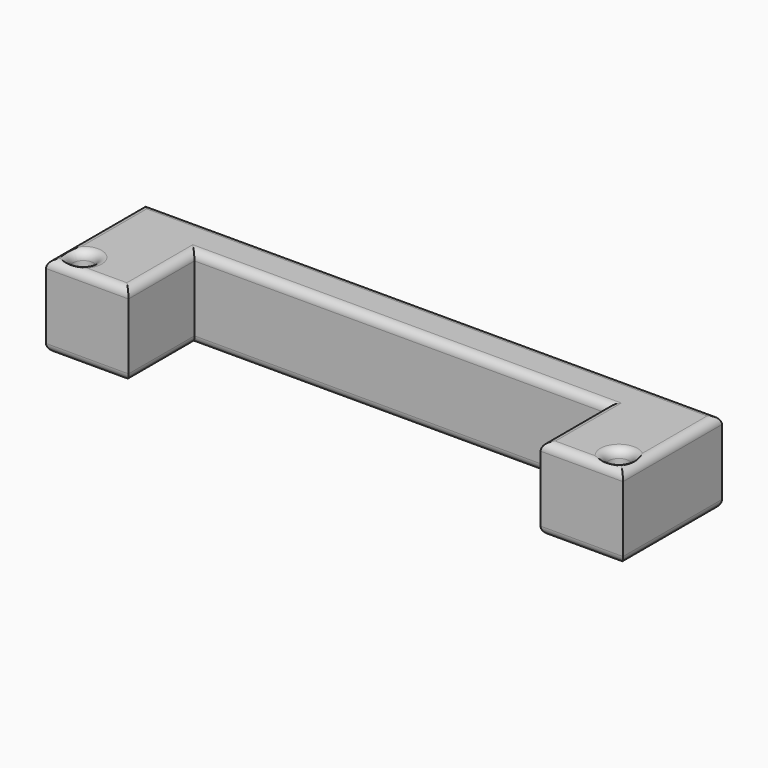
from build123d import *

# Parameters (mm, degrees)
F1_DEPTH     = 20
F3_D         = 5
F5_T1_DEPTH  = 150
F5_T3_DEPTH  = 40
F5_T5_DEPTH  = 30
F5_T7_DEPTH  = 25
F5_T9_DEPTH  = 100
F5_T11_DEPTH = 30
F5_T25_DEPTH = 105
F5_T29_DEPTH = 30
F5_T36_DEPTH = 30
F5_T40_DEPTH = 105
F5_T47_DEPTH = 30
F5_T51_DEPTH = 105
F5_T58_DEPTH = 105
F5_T62_DEPTH = 30


# Not quite as in the source:
# - a fillet or chamfer that OpenCascade refuses, or shapes differently, is made with other operations: its cross-section is extruded or revolved along the edge and cut away or added


with BuildPart() as f1:
    # F0 (on Top) → F1 (new body)
    with BuildSketch(Plane.XY):
        Polygon((0, 30), (0, 20), (50, 20), (50, 0), (70, 0), (70, 30), align=None)
    extrude(amount=F1_DEPTH)

    # F3 (through all)
    with Locations(Plane.XY.offset(20)):
        with Locations((65, 5)):
            Hole(F3_D / 2)

    # F4: F1 across face


with BuildPart() as f1_1:
    add(f1.part)
    add(f1.part.mirror(Plane(origin=(0, 25, 10), x_dir=(0, -1, 0), z_dir=(-1, 0, 0))))

    # F5: fillet of radius 2 on 20 edges, made by hand

    # F5_s2 → F5_t1 (cut)
    with BuildSketch(Plane.YZ.offset(-75)):
        with BuildLine():
            ThreePointArc((30, 18), (29.4142135624, 19.4142135624), (28, 20))
            Line((28, 20), (30, 20))
            Line((30, 20), (30, 18))
        make_face()
        with BuildLine():
            ThreePointArc((30, 2), (29.4142135624, 0.5857864376), (28, 0))
            Line((28, 0), (30, 0))
            Line((30, 0), (30, 2))
        make_face()
    extrude(amount=F5_T1_DEPTH, mode=Mode.SUBTRACT)

    # F5_s4 → F5_t3 (cut)
    with BuildSketch(Plane.XZ.offset(-35)):
        with BuildLine():
            ThreePointArc((-70, 18), (-69.4142135624, 19.4142135624), (-68, 20))
            Line((-68, 20), (-70, 20))
            Line((-70, 20), (-70, 18))
        make_face()
        with BuildLine():
            ThreePointArc((68, 20), (69.4142135624, 19.4142135624), (70, 18))
            Line((70, 18), (70, 20))
            Line((70, 20), (68, 20))
        make_face()
        with BuildLine():
            ThreePointArc((-68, 0), (-69.4142135624, 0.5857864376), (-70, 2))
            Line((-70, 2), (-70, 0))
            Line((-70, 0), (-68, 0))
        make_face()
        with BuildLine():
            ThreePointArc((68, 0), (69.4142135624, 0.5857864376), (70, 2))
            Line((70, 2), (70, 0))
            Line((70, 0), (68, 0))
        make_face()
    extrude(amount=F5_T3_DEPTH, mode=Mode.SUBTRACT)

    # F5_s6 → F5_t5 (cut)
    with BuildSketch(Plane.YZ.offset(-75)):
        with BuildLine():
            ThreePointArc((0, 18), (0.5857864376, 19.4142135624), (2, 20))
            Line((2, 20), (0, 20))
            Line((0, 20), (0, 18))
        make_face()
        with BuildLine():
            ThreePointArc((2, 0), (0.5857864376, 0.5857864376), (0, 2))
            Line((0, 2), (0, 0))
            Line((0, 0), (2, 0))
        make_face()
    extrude(amount=F5_T5_DEPTH, mode=Mode.SUBTRACT)

    # F5_s8 → F5_t7 (cut)
    with BuildSketch(Plane.XZ.offset(-20)):
        with BuildLine():
            ThreePointArc((-50, 18), (-50.5857864376, 19.4142135624), (-52, 20))
            Line((-52, 20), (-50, 20))
            Line((-50, 20), (-50, 18))
        make_face()
        with BuildLine():
            ThreePointArc((50, 18), (50.5857864376, 19.4142135624), (52, 20))
            Line((52, 20), (50, 20))
            Line((50, 20), (50, 18))
        make_face()
        with BuildLine():
            ThreePointArc((-52, 0), (-50.5857864376, 0.5857864376), (-50, 2))
            Line((-50, 2), (-50, 0))
            Line((-50, 0), (-52, 0))
        make_face()
        with BuildLine():
            ThreePointArc((52, 0), (50.5857864376, 0.5857864376), (50, 2))
            Line((50, 2), (50, 0))
            Line((50, 0), (52, 0))
        make_face()
    extrude(amount=F5_T7_DEPTH, mode=Mode.SUBTRACT)

    # F5_s10 → F5_t9 (cut)
    with BuildSketch(Plane.YZ.offset(-50)):
        with BuildLine():
            ThreePointArc((20, 18), (20.5857864376, 19.4142135624), (22, 20))
            Line((22, 20), (20, 20))
            Line((20, 20), (20, 18))
        make_face()
        with BuildLine():
            ThreePointArc((22, 0), (20.5857864376, 0.5857864376), (20, 2))
            Line((20, 2), (20, 0))
            Line((20, 0), (22, 0))
        make_face()
    extrude(amount=F5_T9_DEPTH, mode=Mode.SUBTRACT)

    # F5_s12 → F5_t11 (cut)
    with BuildSketch(Plane.YZ.offset(45)):
        with BuildLine():
            ThreePointArc((0, 18), (0.5857864376, 19.4142135624), (2, 20))
            Line((2, 20), (0, 20))
            Line((0, 20), (0, 18))
        make_face()
        with BuildLine():
            ThreePointArc((2, 0), (0.5857864376, 0.5857864376), (0, 2))
            Line((0, 2), (0, 0))
            Line((0, 0), (2, 0))
        make_face()
    extrude(amount=F5_T11_DEPTH, mode=Mode.SUBTRACT)

    # F5_s13 → F5_t14 (revolve, cut)
    with BuildSketch(Plane.XZ.offset(-5)):
        with BuildLine():
            ThreePointArc((67.5, 18), (68.0857864376, 19.4142135624), (69.5, 20))
            Line((69.5, 20), (67.5, 20))
            Line((67.5, 20), (67.5, 18))
        make_face()
    revolve(axis=Axis((65, 5, 20), (0, 0, 1)), mode=Mode.SUBTRACT)

    # F5_s15 → F5_t16 (revolve, cut)
    with BuildSketch(Plane.XZ.offset(-5)):
        with BuildLine():
            ThreePointArc((-67.5, 18), (-68.0857864376, 19.4142135624), (-69.5, 20))
            Line((-69.5, 20), (-67.5, 20))
            Line((-67.5, 20), (-67.5, 18))
        make_face()
    revolve(axis=Axis((-65, 5, 20), (0, 0, -1)), mode=Mode.SUBTRACT)

    # F5_s17 → F5_t18 (revolve, cut)
    with BuildSketch(Plane.XZ.offset(-5)):
        with BuildLine():
            ThreePointArc((69.5, 0), (68.0857864376, 0.5857864376), (67.5, 2))
            Line((67.5, 2), (67.5, 0))
            Line((67.5, 0), (69.5, 0))
        make_face()
    revolve(axis=Axis((65, 5, 0), (0, 0, 1)), mode=Mode.SUBTRACT)

    # F5_s19 → F5_t20 (revolve, cut)
    with BuildSketch(Plane.XZ.offset(-5)):
        with BuildLine():
            ThreePointArc((-69.5, 0), (-68.0857864376, 0.5857864376), (-67.5, 2))
            Line((-67.5, 2), (-67.5, 0))
            Line((-67.5, 0), (-69.5, 0))
        make_face()
    revolve(axis=Axis((-65, 5, 0), (0, 0, -1)), mode=Mode.SUBTRACT)


with BuildPart() as f5_tool23:
    # F5_s24 → F5_t25 (new body)
    with BuildSketch(Plane.YZ.offset(-55)):
        with BuildLine():
            ThreePointArc((20, 18), (20.5857864376, 19.4142135624), (22, 20))
            Line((22, 20), (20, 20))
            Line((20, 20), (20, 18))
        make_face()
    extrude(amount=F5_T25_DEPTH)

    split(bisect_by=Plane.YZ.offset(-50), keep=Keep.BOTTOM)


with BuildPart() as f5_tool27:
    # F5_s28 → F5_t29 (new body)
    with BuildSketch(Plane.XZ.offset(-25)):
        with BuildLine():
            ThreePointArc((-50, 18), (-50.5857864376, 19.4142135624), (-52, 20))
            Line((-52, 20), (-50, 20))
            Line((-50, 20), (-50, 18))
        make_face()
    extrude(amount=F5_T29_DEPTH)

    split(bisect_by=Plane.XZ.offset(-20), keep=Keep.BOTTOM)


with BuildPart() as f5_tool23_1:
    add(f5_tool23.part)

    # F5_t31: intersect F5_tool27
    add(f5_tool27.part, mode=Mode.INTERSECT)


with BuildPart() as f1_2:
    add(f1_1.part)

    # F5_t21: cut F5_tool23
    add(f5_tool23_1.part, mode=Mode.SUBTRACT)


with BuildPart() as f5_tool34:
    # F5_s35 → F5_t36 (new body)
    with BuildSketch(Plane.XZ.offset(-25)):
        with BuildLine():
            ThreePointArc((50, 18), (50.5857864376, 19.4142135624), (52, 20))
            Line((52, 20), (50, 20))
            Line((50, 20), (50, 18))
        make_face()
    extrude(amount=F5_T36_DEPTH)

    split(bisect_by=Plane.XZ.offset(-20), keep=Keep.BOTTOM)


with BuildPart() as f5_tool38:
    # F5_s39 → F5_t40 (new body)
    with BuildSketch(Plane.YZ.offset(-50)):
        with BuildLine():
            ThreePointArc((20, 18), (20.5857864376, 19.4142135624), (22, 20))
            Line((22, 20), (20, 20))
            Line((20, 20), (20, 18))
        make_face()
    extrude(amount=F5_T40_DEPTH)

    split(bisect_by=Plane.YZ.offset(50), keep=Keep.TOP)


with BuildPart() as f5_tool34_1:
    add(f5_tool34.part)

    # F5_t42: intersect F5_tool38
    add(f5_tool38.part, mode=Mode.INTERSECT)


with BuildPart() as f1_3:
    add(f1_2.part)

    # F5_t32: cut F5_tool34
    add(f5_tool34_1.part, mode=Mode.SUBTRACT)


with BuildPart() as f5_tool45:
    # F5_s46 → F5_t47 (new body)
    with BuildSketch(Plane.XZ.offset(-25)):
        with BuildLine():
            ThreePointArc((-52, 0), (-50.5857864376, 0.5857864376), (-50, 2))
            Line((-50, 2), (-50, 0))
            Line((-50, 0), (-52, 0))
        make_face()
    extrude(amount=F5_T47_DEPTH)

    split(bisect_by=Plane.XZ.offset(-20), keep=Keep.BOTTOM)


with BuildPart() as f5_tool49:
    # F5_s50 → F5_t51 (new body)
    with BuildSketch(Plane.YZ.offset(50)):
        with BuildLine():
            ThreePointArc((22, 0), (20.5857864376, 0.5857864376), (20, 2))
            Line((20, 2), (20, 0))
            Line((20, 0), (22, 0))
        make_face()
    extrude(amount=-F5_T51_DEPTH)

    split(bisect_by=Plane.YZ.offset(-50), keep=Keep.BOTTOM)


with BuildPart() as f5_tool45_1:
    add(f5_tool45.part)

    # F5_t53: intersect F5_tool49
    add(f5_tool49.part, mode=Mode.INTERSECT)


with BuildPart() as f1_4:
    add(f1_3.part)

    # F5_t43: cut F5_tool45
    add(f5_tool45_1.part, mode=Mode.SUBTRACT)


with BuildPart() as f5_tool56:
    # F5_s57 → F5_t58 (new body)
    with BuildSketch(Plane.YZ.offset(55)):
        with BuildLine():
            ThreePointArc((22, 0), (20.5857864376, 0.5857864376), (20, 2))
            Line((20, 2), (20, 0))
            Line((20, 0), (22, 0))
        make_face()
    extrude(amount=-F5_T58_DEPTH)

    split(bisect_by=Plane.YZ.offset(50), keep=Keep.TOP)


with BuildPart() as f5_tool60:
    # F5_s61 → F5_t62 (new body)
    with BuildSketch(Plane.XZ.offset(-25)):
        with BuildLine():
            ThreePointArc((52, 0), (50.5857864376, 0.5857864376), (50, 2))
            Line((50, 2), (50, 0))
            Line((50, 0), (52, 0))
        make_face()
    extrude(amount=F5_T62_DEPTH)

    split(bisect_by=Plane.XZ.offset(-20), keep=Keep.BOTTOM)


with BuildPart() as f5_tool56_1:
    add(f5_tool56.part)

    # F5_t64: intersect F5_tool60
    add(f5_tool60.part, mode=Mode.INTERSECT)


with BuildPart() as f1_5:
    add(f1_4.part)

    # F5_t54: cut F5_tool56
    add(f5_tool56_1.part, mode=Mode.SUBTRACT)


solid = f1_5.part
